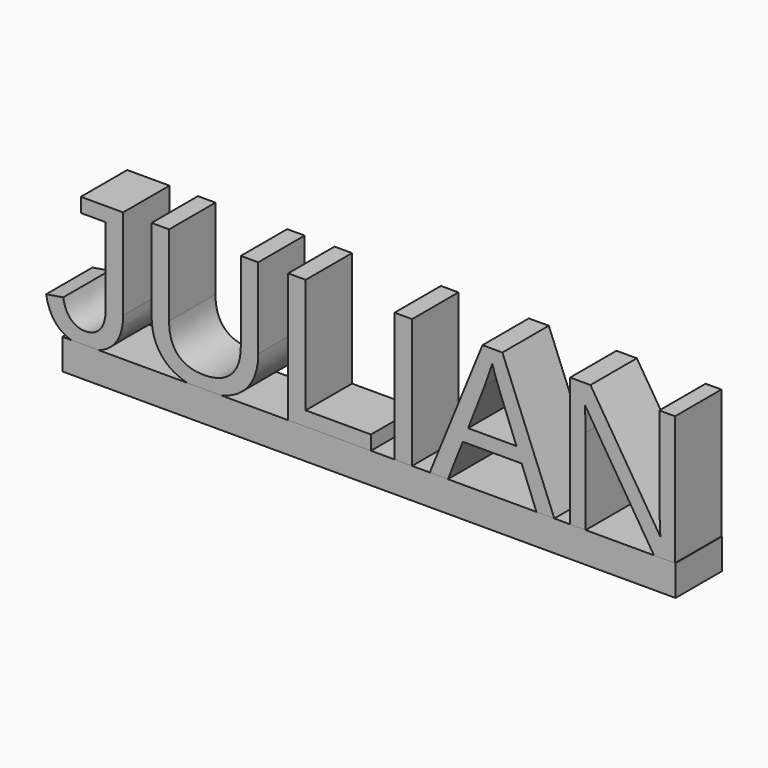
from build123d import *

# Parameters (mm, degrees)
F0_TEXT_SIZE = 61.7361111111
F1_DEPTH     = 19.05
F2_W         = 201.5417665243
F2_H         = 10.0486492738
F3_DEPTH     = 19.05


# Not quite as in the source:
# - Text() gives the source's letters only with a copy of the font that has no kerning and outlines rounded to 1/6400 em; it was checked with that copy


with BuildPart() as f1:
    # F0 (on Front) → F1 (new body)
    with BuildSketch(Plane.XZ):
        with Locations((-82.7182041448, 0)):
            Text('JULIAN', F0_TEXT_SIZE, font='Arimo', text_align=(TextAlign.LEFT, TextAlign.BOTTOM))
    extrude(amount=F1_DEPTH)


with BuildPart() as f3:
    # F2 (on Front) → F3 (new body)
    with BuildSketch(Plane.XZ):
        with Locations((24.3456885219, -5.0243246369)):
            Rectangle(F2_W, F2_H)
    extrude(amount=F3_DEPTH)


solid = Compound([f1.part, f3.part])
